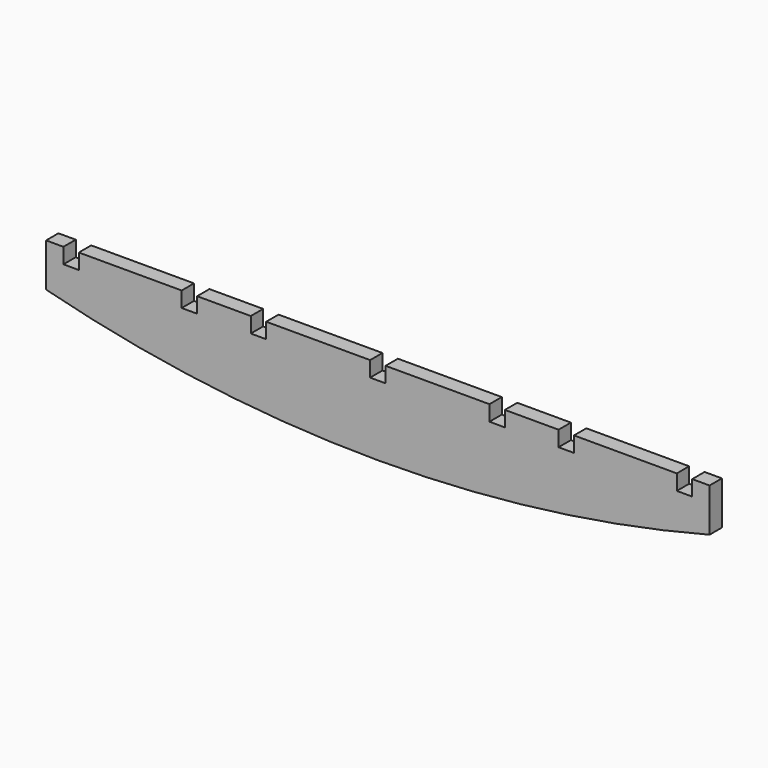
from build123d import *

# Parameters (mm, degrees)
F1_DEPTH = 4.45


# Not quite as in the source:
# - ends of sketch curves that miss each other by under 0.0002 mm in the source are joined


with BuildPart() as f1:
    # F0 (on Front) → F1 (new body)
    with BuildSketch(Plane.XZ):
        with BuildLine():
            Line((2.225, 93.35), (2.225, 88.9))
            Line((2.225, 88.9), (-2.225, 88.9))
            Line((-2.225, 88.9), (-2.225, 93.35))
            Line((-2.225, 93.35), (-32.1837038577, 93.35))
            Line((-32.1837038577, 93.35), (-32.1837038577, 88.9))
            Line((-32.1837038577, 88.9), (-36.6337038577, 88.9))
            Line((-36.6337038577, 88.9), (-36.6337038577, 93.35))
            Line((-36.6337038577, 93.35), (-52.1105349839, 93.35))
            Line((-52.1105349839, 93.35), (-52.1105349839, 88.9))
            Line((-52.1105349839, 88.9), (-56.5605349839, 88.9))
            Line((-56.5605349839, 88.9), (-56.5605349839, 93.35))
            Line((-56.5605349839, 93.35), (-86.2080463052, 93.35))
            Line((-86.2080463052, 93.35), (-86.2080463052, 88.9))
            Line((-86.2080463052, 88.9), (-90.6580463052, 88.9))
            Line((-90.6580463052, 88.9), (-90.6580463052, 93.35))
            Line((-90.6580463052, 93.35), (-95.6580463052, 93.35))
            Line((-95.6580463052, 93.35), (-95.6580463052, 80.85))
            ThreePointArc((-95.6580463052, 80.85), (0, 68.6427723395), (95.6580463052, 80.85))
            Line((95.6580463052, 80.85), (95.6580463052, 93.35))
            Line((95.6580463052, 93.35), (90.6580463052, 93.35))
            Line((90.6580463052, 93.35), (90.6580454826, 88.9))
            Line((90.6580454826, 88.9), (86.2080454826, 88.9))
            Line((86.2080454826, 88.9), (86.2080454826, 93.35))
            Line((86.2080454826, 93.35), (56.5605341613, 93.35))
            Line((56.5605341613, 93.35), (56.5605341613, 88.9))
            Line((56.5605341613, 88.9), (52.1105341613, 88.9))
            Line((52.1105341613, 88.9), (52.1105341613, 93.35))
            Line((52.1105341613, 93.35), (36.6337030351, 93.35))
            Line((36.6337030351, 93.35), (36.6337030351, 88.9))
            Line((36.6337030351, 88.9), (32.1837030351, 88.9))
            Line((32.1837030351, 88.9), (32.1837030351, 93.35))
            Line((32.1837030351, 93.35), (2.225, 93.35))
        make_face()
    extrude(amount=F1_DEPTH)


solid = f1.part
